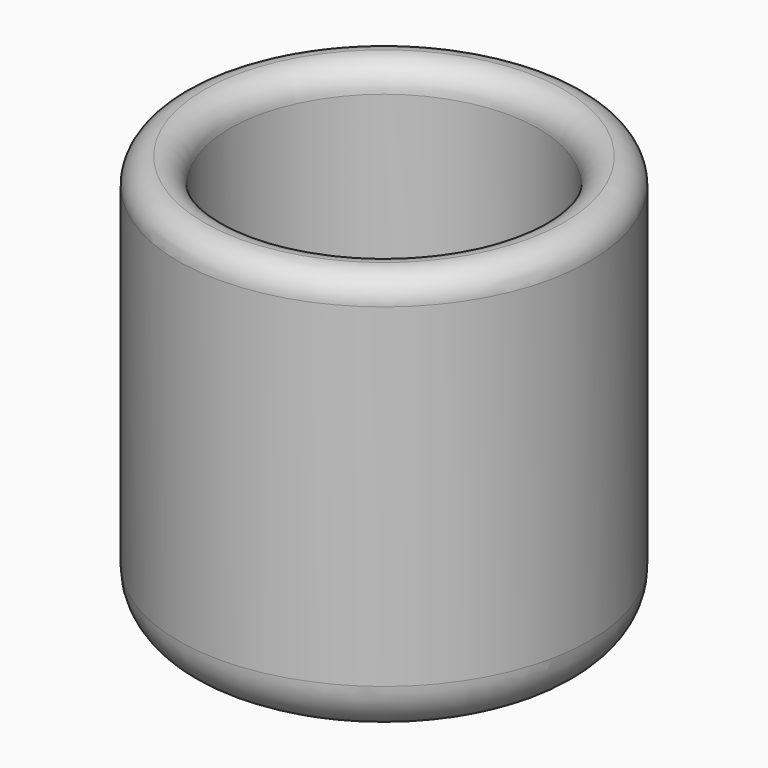
from build123d import *

# Parameters (mm, degrees)
F0_R     = 25.4
F1_DEPTH = 50.8
F2_R     = 19.05
F3_DEPTH = 44.45
F4_R     = 3.17499
F5_R     = 12.7
F6_R     = 6.35


# Not quite as in the source:
# - a fillet or chamfer is up to 0.001 mm smaller than in the source, because OpenCascade refuses the exact size


with BuildPart() as f1:
    # F0 (on Top) → F1 (new body)
    with BuildSketch(Plane.XY):
        Circle(F0_R)
    extrude(amount=F1_DEPTH)

    # F2 (on face) → F3 (cut)
    with BuildSketch(Plane.XY.offset(50.8)):
        Circle(F2_R)
    extrude(amount=-F3_DEPTH, mode=Mode.SUBTRACT)

    # F4 (radius 3.175 in the source; OpenCascade refuses exactly that, so slightly less here)
    f4_edges = [f1.edges().sort_by_distance(p)[0] for p in [
        (-25.4, 0, 50.8),
        (-19.05, 0, 50.8),
    ]]
    fillet(f4_edges, radius=F4_R)

    # F5
    f5_edges = [f1.edges().sort_by_distance(p)[0] for p in [
        (-19.05, 0, 6.35),
    ]]
    fillet(f5_edges, radius=F5_R)

    # F6
    f6_edges = [f1.edges().sort_by_distance(p)[0] for p in [
        (-25.4, 0, 0),
    ]]
    fillet(f6_edges, radius=F6_R)


solid = f1.part
